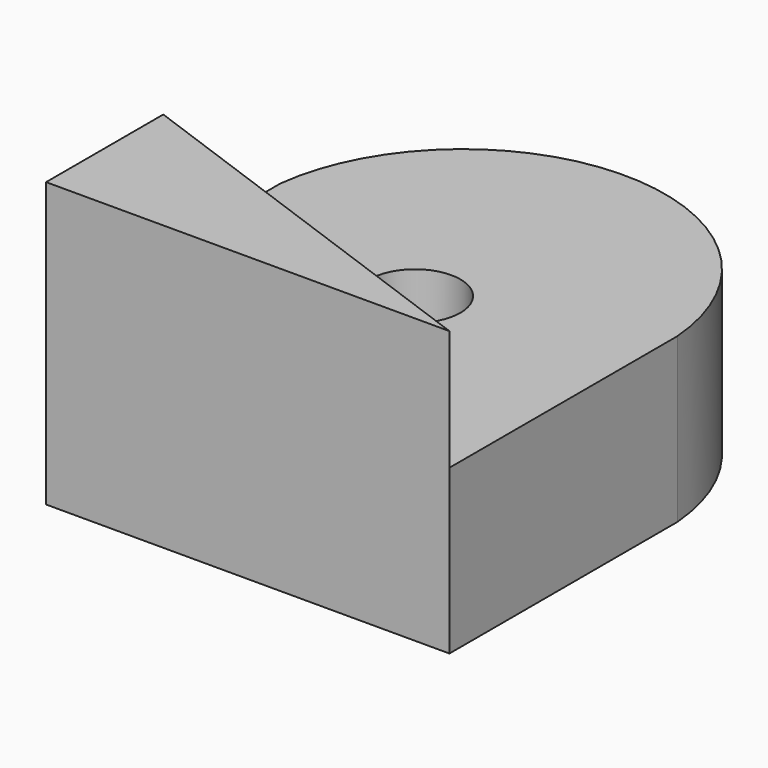
from build123d import *

# Parameters (mm, degrees)
F1_DEPTH = 59.944
F0_R     = 9.5854875755
F2_DEPTH = 34.544


with BuildPart() as f1:
    # F0 (on Top) → F1 (new body)
    with BuildSketch(Plane.XY):
        Polygon((42.7391566336, -44.3220846355), (-42.4513481557, -13.3829666302), (-42.4513481557, -44.3220846355), align=None)
    extrude(amount=F1_DEPTH)

    # F0 (on Top) → F2 (join)
    with BuildSketch(Plane.XY):
        with BuildLine():
            ThreePointArc((42.7391566336, 15.8293172717), (0.9256115544, 55.2569720027), (-42.4513481557, 17.5561513752))
            Line((-42.4513481557, 17.5561513752), (-42.4513481557, -13.3829666302))
            Line((-42.4513481557, -13.3829666302), (42.7391566336, -44.3220846355))
            Line((42.7391566336, -44.3220846355), (42.7391566336, 15.8293172717))
        make_face()
        Circle(F0_R, mode=Mode.SUBTRACT)
    extrude(amount=F2_DEPTH)


solid = f1.part
